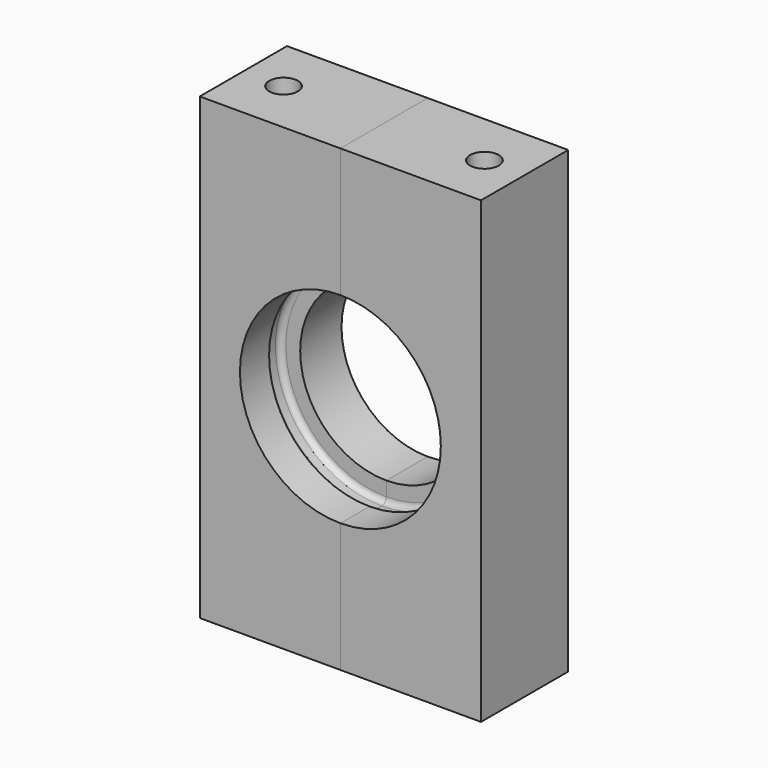
from build123d import *
from build123d import SkipClean  # not in build123d's __all__

# Parameters (mm, degrees)
F0_W     = 24.5
F0_H     = 80
F1_DEPTH = 9.5
F3_D     = 5
F3_DEPTH = 22
F3_TIP   = 1.5021515476
F5_D     = 7
F5_DEPTH = 22
F5_TIP   = 2.1030121666
F7_ANGLE = 180


with BuildPart() as f1:
    # F0 (on Front) → F1 (new body, symmetric)
    with BuildSketch(Plane.XZ):
        with Locations((12.25, 0)):
            Rectangle(F0_W, F0_H)
    extrude(amount=F1_DEPTH, both=True)

    # F3
    with Locations(Plane.XY.offset(40)):
        with Locations((17.5, 0)):
            Hole(F3_D / 2, depth=F3_DEPTH)
            with Locations((0, 0, -(F3_DEPTH + F3_TIP / 2))):  # 118° drill point
                Cone(0, F3_D / 2, F3_TIP, mode=Mode.SUBTRACT)

    # F5
    with Locations(Plane(origin=(0, 0, -40), x_dir=(1, 0, 0), z_dir=(0, 0, -1))):
        with Locations((15, 0)):
            Hole(F5_D / 2, depth=F5_DEPTH)
            with Locations((0, 0, -(F5_DEPTH + F5_TIP / 2))):  # 118° drill point
                Cone(0, F5_D / 2, F5_TIP, mode=Mode.SUBTRACT)

    # F6 (on Right) → F7 (revolve, cut)
    with BuildSketch(Plane.YZ):
        with BuildLine():
            Line((-9.5, 0), (9.5, 0))
            Line((9.5, 0), (9.5, 15))
            Line((9.5, 15), (0.5, 15))
            Line((0.5, 15), (0.5, 17.5))
            ThreePointArc((0.5, 17.5), (0.2071067812, 18.2071067812), (-0.5, 18.5))
            Line((-0.5, 18.5), (-2, 18.5))
            ThreePointArc((-2, 18.5), (-2.5, 18.3660254038), (-2.8660254038, 18))
            Line((-2.8660254038, 18), (-3.1547005384, 17.5))
            Line((-3.1547005384, 17.5), (-9.5, 17.5))
            Line((-9.5, 17.5), (-9.5, 0))
        make_face()
    revolve(axis=Axis((0, 0, 0), (0, 1, 0)), revolution_arc=F7_ANGLE, mode=Mode.SUBTRACT)

    # F8: F1 across plane


with BuildPart() as f1_1:
    add(f1.part, clean=False)
    with SkipClean():  # cleaning this boolean's faces spoils the solid; the shape is the same uncleaned
        add(f1.part.mirror(Plane.YZ), clean=False)


solid = f1_1.part
